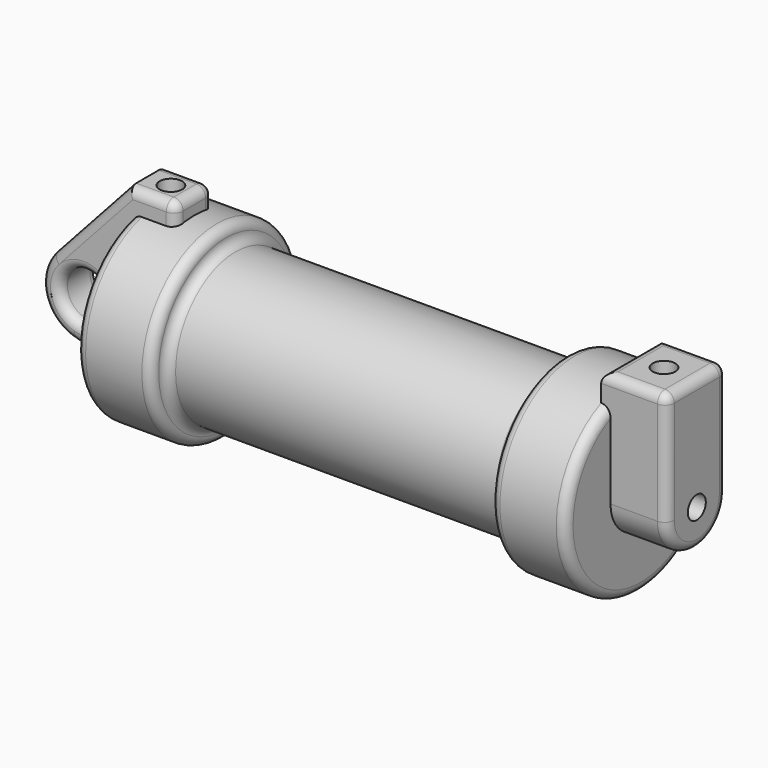
from build123d import *

# Parameters (mm, degrees)
F0_W      = 5.842
F0_H      = 12.7
F0_R      = 3.175
F1_DEPTH  = 3.175
F3_R      = 1.524
F4_DEPTH  = 7.62
F5_DEPTH  = 1.27
F6_DEPTH  = 56.134
F7_R      = 1.524
F8_DEPTH  = 17.78
F9_R      = 1.524
F10_DEPTH = 10.414
F11_R     = 1.26999
F11_2_R   = 1.26999


# Not quite as in the source:
# - a fillet or chamfer is up to 0.001 mm smaller than in the source, because OpenCascade refuses the exact size


with BuildPart() as f1:
    # F0 (on Front) → F1 (new body, symmetric)
    with BuildSketch(Plane.XZ):
        with BuildLine():
            Line((-0.9398, 0), (0, 0))
            Line((0, 0), (0, 12.7))
            Line((0, 12.7), (5.842, 12.7))
            Line((5.842, 12.7), (5.842, 15.24))
            Line((5.842, 15.24), (-0.508, 15.24))
            Line((-0.508, 15.24), (-10.8806298187, 3.8475430269))
            ThreePointArc((-10.8806298187, 3.8475430269), (-4.5919612295, 5.3297205562), (-0.9398, 0))
        make_face()
        with Locations((2.921, 6.35)):
            Rectangle(F0_W, F0_H)
        with BuildLine():
            Line((5.842, 0), (0, 0))
            Line((0, 0), (-0.9398, 0))
            ThreePointArc((-0.9398, 0), (-3.1957909266, -4.5493385486), (-8.1826630726, -5.5069827884))
            Line((-8.1826630726, -5.5069827884), (5.842, -9.398))
            Line((5.842, -9.398), (5.842, 0))
        make_face()
        with BuildLine():
            ThreePointArc((-8.1826630726, -5.5069827884), (-3.1957909266, -4.5493385486), (-0.9398, 0))
            ThreePointArc((-0.9398, 0), (-4.5919612295, 5.3297205562), (-10.8806298187, 3.8475430269))
            ThreePointArc((-10.8806298187, 3.8475430269), (-12.1459778134, -1.5837270034), (-8.1826630726, -5.5069827884))
        make_face()
        with Locations((-6.6548, 0)):
            Circle(F0_R, mode=Mode.SUBTRACT)
    extrude(amount=F1_DEPTH, both=True)

    # F7 (on face) → F8 (cut)
    with BuildSketch(Plane.XY.offset(15.24)):
        with Locations((2.667, 0)):
            Circle(F7_R)
    extrude(amount=-F8_DEPTH, mode=Mode.SUBTRACT)

    # F11 (radius 1.27 in the source; OpenCascade refuses exactly that, so slightly less here)
    f11_edges = [f1.edges().sort_by_distance(p)[0] for p in [
        (-1.170332, -3.175, -7.452491),
        (5.842, -3.175, 2.921),
        (2.667, -3.175, 15.24),
        (-5.694315, -3.175, 9.543772),
        (-12.145978, -3.175, -1.583727),
        (-9.8298, -3.175, 0),
        (-1.170332, 3.175, -7.452491),
        (5.842, 3.175, 2.921),
        (2.667, 3.175, 15.24),
        (-5.694315, 3.175, 9.543772),
        (-12.145978, 3.175, -1.583727),
        (-9.8298, 3.175, 0),
        (5.842, 0, 15.24),
    ]]
    fillet(f11_edges, radius=F11_R)


with BuildPart() as f2:
    # F0 (on Front) → F2 (revolve)
    with BuildSketch(Plane.XZ):
        Polygon((5.842, 12.7), (5.842, 0), (66.294, 0), (66.294, 12.7), (56.134, 12.7), (56.134, 10.16), (10.16, 10.16), (10.16, 12.7), align=None)
        with Locations((2.921, 6.35)):
            Rectangle(F0_W, F0_H)
    revolve(axis=Axis((33.147, 0, 0), (-1, 0, 0)))

    # F3 (on face) → F4 (join)
    with BuildSketch(Plane.YZ.offset(66.294)):
        with BuildLine():
            ThreePointArc((-5.08, 0), (0, 5.08), (5.08, 0))
            Line((5.08, 0), (5.08, 11.6397422652))
            ThreePointArc((5.08, 11.6397422652), (0, 12.7), (-5.08, 11.6397422652))
            Line((-5.08, 11.6397422652), (-5.08, 0))
        make_face()
        with BuildLine():
            ThreePointArc((-5.08, 0), (0, -5.08), (5.08, 0))
            ThreePointArc((5.08, 0), (0, 5.08), (-5.08, 0))
        make_face()
        Circle(F3_R, mode=Mode.SUBTRACT)
        with BuildLine():
            ThreePointArc((-5.08, 11.6397422652), (0, 12.7), (5.08, 11.6397422652))
            Line((5.08, 11.6397422652), (5.08, 15.24))
            Line((5.08, 15.24), (-5.08, 15.24))
            Line((-5.08, 15.24), (-5.08, 11.6397422652))
        make_face()
    extrude(amount=F4_DEPTH)

    # F5 (add): a face of the model
    f5_faces = [f2.faces().sort_by_distance(p)[0] for p in [
        (66.294, 0, 13.7792682875),
    ]]
    extrude(f5_faces, amount=F5_DEPTH)

    # F6 (cut, through all): a face of the model
    f6_faces = [f2.faces().sort_by_distance(p)[0] for p in [
        (66.294, 0, 0),
    ]]
    extrude(f6_faces, amount=-F6_DEPTH, mode=Mode.SUBTRACT)

    # F9 (on face) → F10 (cut)
    with BuildSketch(Plane.XY.offset(15.24)):
        with Locations((69.469, 0)):
            Circle(F9_R)
    extrude(amount=-F10_DEPTH, mode=Mode.SUBTRACT)

    # F11#2 (radius 1.27 in the source; OpenCascade refuses exactly that, so slightly less here)
    f11_2_edges = [f2.edges().sort_by_distance(p)[0] for p in [
        (56.134, 0, -10.16),
        (10.16, 0, -10.16),
        (33.147, 0, 10.16),
        (10.16, 0, -12.7),
        (0, 0, -12.7),
        (5.08, 0, 12.7),
        (66.294, 0, -12.7),
        (56.134, 0, -12.7),
        (73.914, 0, -5.08),
        (73.914, 5.08, 7.62),
        (73.914, -5.08, 7.62),
        (69.469, 5.08, 15.24),
        (73.914, 0, 15.24),
        (65.024, 0, 15.24),
        (69.469, -5.08, 15.24),
    ]]
    fillet(f11_2_edges, radius=F11_2_R)


solid = Compound([f1.part, f2.part])
